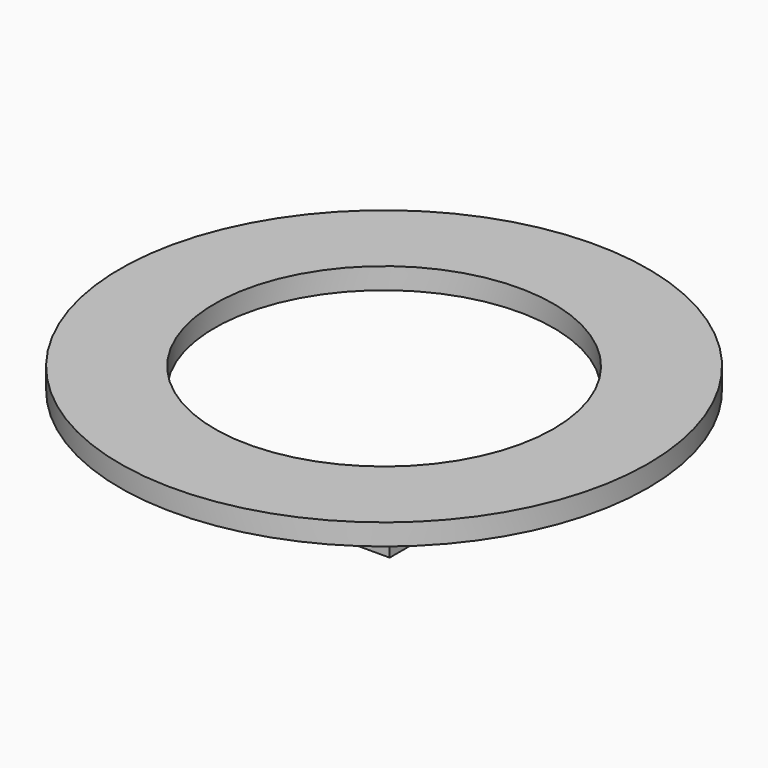
from build123d import *

# Parameters (mm, degrees)
F1_W     = 25.3329826519
F1_H     = 3.7999469787
F2_DEPTH = 12.7
F0_R     = 78.9653812796
F0_R_2   = 50.6914401609
F5_DEPTH = 6.35


# Not quite as in the source:
# - the program builds the solid bodies; features that only make, move or delete a surface that nothing else refers to are left out


with BuildPart() as f2:
    # F1 (on Front) → F2 (new body, symmetric)
    with BuildSketch(Plane.XZ):
        with Locations((-0.8444325067, -33.1439850852)):
            Rectangle(F1_W, F1_H)
    extrude(amount=F2_DEPTH, both=True)


with BuildPart() as f5:
    # F0 (on Top) → F5 (new body)
    with BuildSketch(Plane.XY):
        Circle(F0_R)
        Circle(F0_R_2, mode=Mode.SUBTRACT)
    extrude(amount=F5_DEPTH)


solid = Compound([f2.part, f5.part])
